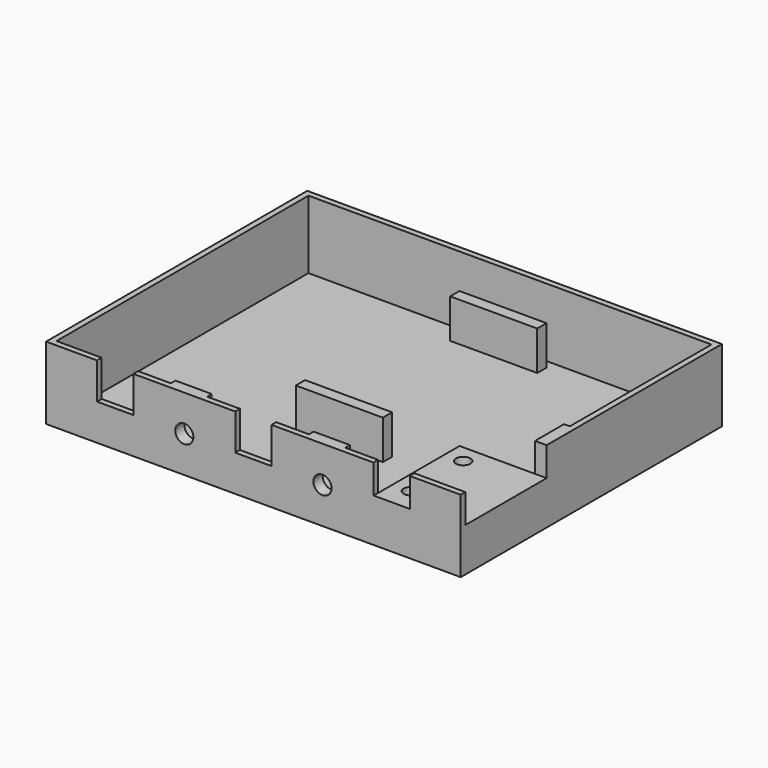
from build123d import *

# Parameters (mm, degrees)
F0_W     = 12
F0_H     = 1.6
F0_H_2   = 7
F0_R     = 1
F1_DEPTH = 0.6
F2_W     = 12
F2_H     = 1.6
F2_H_2   = 7
F2_R     = 1
F3_DEPTH = 5.4
F4_W     = 2.5
F4_H     = 0.8
F4_W_2   = 0.8
F4_H_2   = 5
F5_DEPTH = 9.4
F6_DEPTH = 4.4
F7_DEPTH = 1
F8_R     = 1.25
F9_DEPTH = 1.6


# Not quite as in the source:
# - a feature names something its author has since deleted; it is built from what else it names


with BuildPart() as f1:
    # F0 (on Top) → F1 (new body)
    with BuildSketch(Plane.XY):
        Polygon((-57.15, 0), (-12, 0), (-12, 7), (-12, 14), (0, 14), (0, 43), (-22.575, 43), (-22.575, 41.4), (-34.575, 41.4), (-34.575, 43), (-57.15, 43), align=None)
        with Locations((-28.575, 15.6)):
            Rectangle(F0_W, F0_H, mode=Mode.SUBTRACT)
        Polygon((-57.15, 45), (-57.15, 43), (-34.575, 43), (-22.575, 43), (0, 43), (0, 45), align=None)
        with Locations((-6, 10.5)):
            Rectangle(F0_W, F0_H_2)
        with Locations((-9.5, 11.5)):
            Circle(F0_R, mode=Mode.SUBTRACT)
        with Locations((-6, 3.5)):
            Rectangle(F0_W, F0_H_2)
        with Locations((-9.5, 2.5)):
            Circle(F0_R, mode=Mode.SUBTRACT)
        with Locations((-28.575, 42.2)):
            Rectangle(F0_W, F0_H)
        with Locations((-28.575, 15.6)):
            Rectangle(F0_W, F0_H)
        with Locations((-9.5, 11.5)):
            Circle(F0_R)
        with Locations((-9.5, 2.5)):
            Circle(F0_R)
    extrude(amount=F1_DEPTH)

    # F2 (on face) → F3 (join)
    with BuildSketch(Plane.XY.offset(0.6)):
        with Locations((-28.575, 42.2)):
            Rectangle(F2_W, F2_H)
        with Locations((-28.575, 15.6)):
            Rectangle(F2_W, F2_H)
        with Locations((-6, 11.3)):
            Rectangle(F2_W, F2_H_2)
        with Locations((-9.5, 12.3)):
            Circle(F2_R, mode=Mode.SUBTRACT)
        with Locations((-6, 4.3)):
            Rectangle(F2_W, F2_H_2)
        with Locations((-9.5, 3.3)):
            Circle(F2_R, mode=Mode.SUBTRACT)
    extrude(amount=F3_DEPTH)

    # F4 (on face) → F5 (join)
    with BuildSketch(Plane.XY.offset(0.6)):
        Polygon((-45.125, 0.8), (-45.125, 0), (-31.075, 0), (-31.075, 0.8), (-35.6, 0.8), (-38.1, 0.8), (-40.6, 0.8), align=None)
        with Locations((-36.85, 1.2)):
            Rectangle(F4_W, F4_H)
        with Locations((-39.35, 1.2)):
            Rectangle(F4_W, F4_H)
        Polygon((-21.55, 1.6), (-21.55, 0.8), (-16.55, 0.8), (-16.55, 1.6), (-19.05, 1.6), align=None)
        Polygon((-26.075, 0.8), (-26.075, 0), (-12.025, 0), (-12.025, 0.8), (-16.55, 0.8), (-21.55, 0.8), align=None)
        Polygon((0, 0), (0, 0.8), (-0.8, 0.8), (-7.025, 0.8), (-7.025, 0), align=None)
        Polygon((0, 45), (-57.15, 45), (-57.15, 0), (-50.125, 0), (-50.125, 0.8), (-56.35, 0.8), (-56.35, 44.2), (-0.8, 44.2), (-0.8, 19.8), (-0.8, 14.8), (0, 14.8), align=None)
        with Locations((-1.2, 17.3)):
            Rectangle(F4_W_2, F4_H_2)
    extrude(amount=F5_DEPTH)

    # F4 (on face) → F6 (join)
    with BuildSketch(Plane.XY.offset(0.6)):
        Polygon((-31.075, 0.8), (-31.075, 0), (-26.075, 0), (-26.075, 0.8), (-28.575, 0.8), align=None)
        Polygon((-50.125, 0.8), (-50.125, 0), (-45.125, 0), (-45.125, 0.8), (-47.625, 0.8), align=None)
        Polygon((-12.025, 0), (-7.025, 0), (-7.025, 0.8), (-9.525, 0.8), (-12, 0.8), (-12.025, 0.8), align=None)
    extrude(amount=F6_DEPTH)

    # F7 (add): a face of the model
    f7_faces = [f1.faces().sort_by_distance(p)[0] for p in [
        (-9.525, 0.4, 5),
    ]]
    extrude(f7_faces, amount=F7_DEPTH)

    # F8 (on face) → F9 (cut)
    with BuildSketch(Plane.XZ):
        with Locations((-38.1, 5)):
            Circle(F8_R)
        with BuildLine():
            ThreePointArc((-17.8, 5), (-18.1661165235, 5.8838834765), (-19.05, 6.25))
            ThreePointArc((-19.05, 6.25), (-19.9338834765, 4.1161165235), (-17.8, 5))
        make_face()
    extrude(amount=-F9_DEPTH, mode=Mode.SUBTRACT)


solid = f1.part
